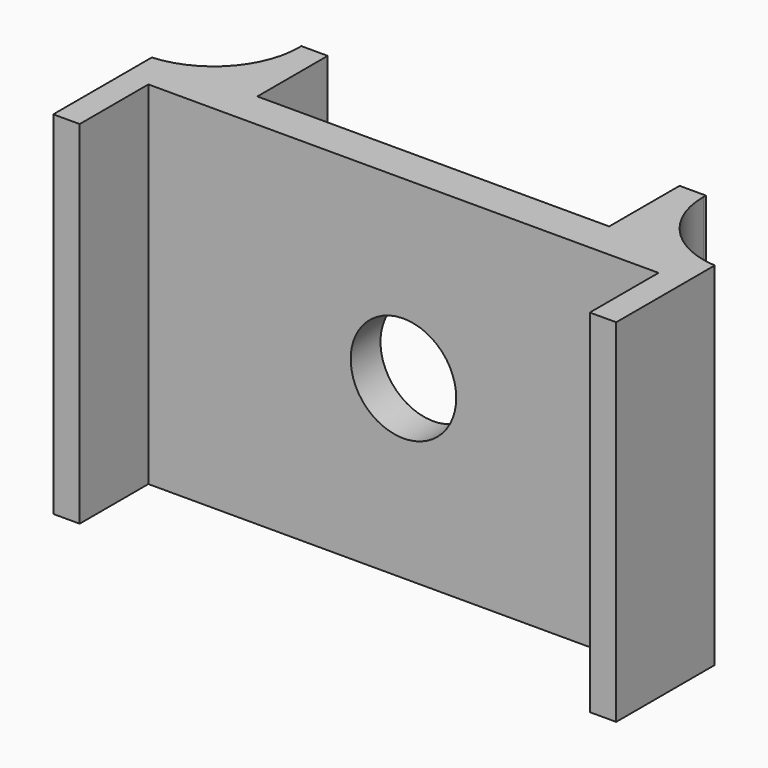
from build123d import *

# Parameters (mm, degrees)
F1_DEPTH    = 20
F2_T1_DEPTH = 20
F3_R        = 3
F4_DEPTH    = 25


# Not quite as in the source:
# - a fillet or chamfer that OpenCascade refuses, or shapes differently, is made with other operations: its cross-section is extruded or revolved along the edge and cut away or added


with BuildPart() as f1:
    # F0 (on Top) → F1 (new body)
    with BuildSketch(Plane.XY):
        Polygon((0, -7), (0, 0), (-4.5, 0), (-4.5, 5), (-6, 5), (-6, 0), (-26, 0), (-26, 5), (-27.5, 5), (-27.5, 0), (-32, 0), (-32, -7), (-30.5, -7), (-30.5, -2.1179924456), (-1.5, -2.1179924456), (-1.5, -7), align=None)
    extrude(amount=F1_DEPTH)

    # F2: fillet of radius 4.8260129112 on 2 edges, made by hand

    # F2_s2 → F2_t1 (join)
    with BuildSketch(Plane.XY):
        with BuildLine():
            ThreePointArc((-27.5, 4.814988702), (-28.8001269844, 1.5197604777), (-32, 0))
            Line((-32, 0), (-27.5, 0))
            Line((-27.5, 0), (-27.5, 4.814988702))
        make_face()
        with BuildLine():
            ThreePointArc((0, 0), (-3.1998730156, 1.5197604777), (-4.5, 4.814988702))
            Line((-4.5, 4.814988702), (-4.5, 0))
            Line((-4.5, 0), (0, 0))
        make_face()
    extrude(amount=F2_T1_DEPTH)

    # F3 (on face) → F4 (cut)
    with BuildSketch(Plane.XZ.offset(2.1179924456)):
        with Locations((-16, 10)):
            Circle(F3_R)
    extrude(amount=-F4_DEPTH, mode=Mode.SUBTRACT)


solid = f1.part
